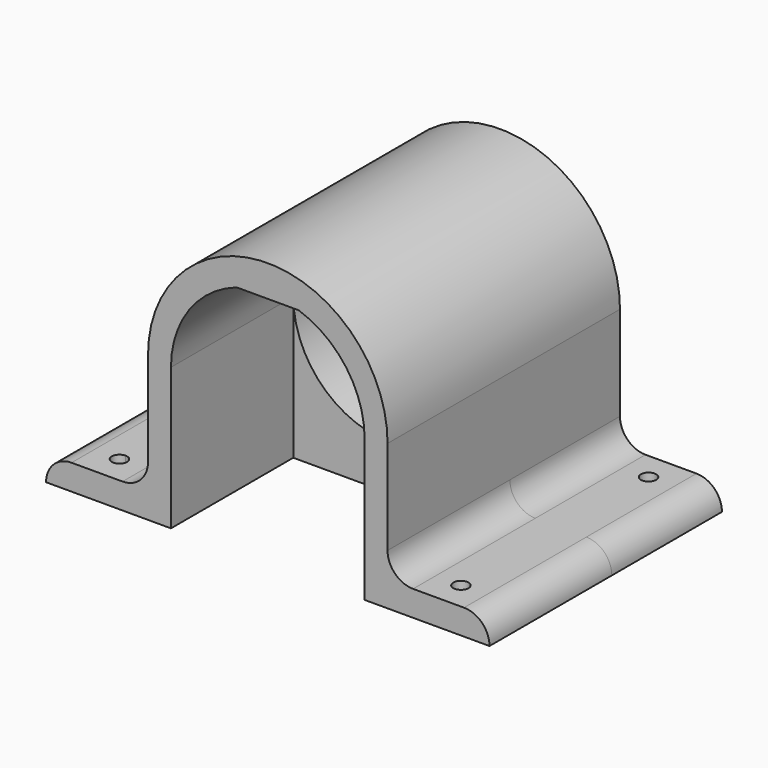
from build123d import *

# Parameters (mm, degrees)
F1_DEPTH  = 2
F2_R      = 1.5
F3_DEPTH  = 5
F4_R      = 19
F5_DEPTH  = 27
F6_W      = 47
F6_H      = 27
F7_DEPTH  = 5
F8_W      = 27
F8_H      = 5
F9_DEPTH  = 20
F10_W     = 27
F10_H     = 5
F11_DEPTH = 20
F12_R     = 4.99999
F14_DEPTH = 30
F16_DEPTH = 4
F18_DEPTH = 25


# Not quite as in the source:
# - a fillet or chamfer is up to 0.001 mm smaller than in the source, because OpenCascade refuses the exact size


with BuildPart() as f1:
    # F0 (on Front) → F1 (new body)
    with BuildSketch(Plane.XZ):
        with BuildLine():
            Line((-23.5, -23.5), (0, -23.5))
            Line((0, -23.5), (23.5, -23.5))
            Line((23.5, -23.5), (23.5, 0))
            ThreePointArc((23.5, 0), (0, 23.5), (-23.5, 0))
            Line((-23.5, 0), (-23.5, -23.5))
        make_face()
    extrude(amount=F1_DEPTH)

    # F2 (on face) → F3 (cut)
    with BuildSketch(Plane.XZ.offset(2)):
        with Locations((15.5, 0)):
            Circle(F2_R)
        with Locations((7.75, 13.4233937587)):
            Circle(F2_R)
        with Locations((-7.75, 13.4233937587)):
            Circle(F2_R)
        with Locations((-15.5, 0)):
            Circle(F2_R)
        with Locations((-7.75, -13.4233937587)):
            Circle(F2_R)
        with Locations((7.75, -13.4233937587)):
            Circle(F2_R)
        with BuildLine():
            Line((6.5, -7), (6.5, 7))
            ThreePointArc((6.5, 7), (0, 13.5), (-6.5, 7))
            Line((-6.5, 7), (-6.5, -7))
            ThreePointArc((-6.5, -7), (0, -13.5), (6.5, -7))
        make_face()
    extrude(amount=-F3_DEPTH, mode=Mode.SUBTRACT)

    # F4 (on Front) → F5 (join)
    with BuildSketch(Plane.XZ):
        with BuildLine():
            ThreePointArc((23.5, 0), (0, 23.5), (-23.5, 0))
            Line((-23.5, 0), (-23.5, -23.5))
            Line((-23.5, -23.5), (23.5, -23.5))
            Line((23.5, -23.5), (23.5, 0))
        make_face()
        with Locations((0, -0.6784388353)):
            Circle(F4_R, mode=Mode.SUBTRACT)
    extrude(amount=F5_DEPTH)

    # F6 (on face) → F7 (join)
    with BuildSketch(Plane(origin=(0, 0, -23.5), x_dir=(1, 0, 0), z_dir=(0, 0, -1))):
        with Locations((0, 13.5)):
            Rectangle(F6_W, F6_H)
    extrude(amount=F7_DEPTH)

    # F8 (on face) → F9 (join)
    with BuildSketch(Plane(origin=(-23.5, 0, 0), x_dir=(0, -1, 0), z_dir=(-1, 0, 0))):
        with Locations((13.5, -26)):
            Rectangle(F8_W, F8_H)
    extrude(amount=F9_DEPTH)

    # F10 (on face) → F11 (join)
    with BuildSketch(Plane.YZ.offset(23.5)):
        with Locations((-13.5, -26)):
            Rectangle(F10_W, F10_H)
    extrude(amount=F11_DEPTH)

    # F12 (radius 5 in the source; OpenCascade refuses exactly that, so slightly less here)
    f12_edges = [f1.edges().sort_by_distance(p)[0] for p in [
        (23.5, -13.5, -23.5),
        (43.5, -13.5, -23.5),
        (-23.5, -13.5, -23.5),
        (-43.5, -13.5, -23.5),
    ]]
    fillet(f12_edges, radius=F12_R)

    # F13 (on face) → F14 (join)
    with BuildSketch(Plane.XZ.offset(27)):
        with BuildLine():
            Line((23.5, -18.5), (23.5, 0))
            ThreePointArc((23.5, 0), (0, 23.5), (-23.5, 0))
            Line((-23.5, 0), (-23.5, -18.5))
            ThreePointArc((-23.5, -18.5), (-24.9644660941, -22.0355339059), (-28.5, -23.5))
            Line((-28.5, -23.5), (-38.5, -23.5))
            ThreePointArc((-38.5, -23.5), (-42.0355339059, -24.9644660941), (-43.5, -28.5))
            Line((-43.5, -28.5), (-19, -28.5))
            Line((-19, -28.5), (-19, -0.6784388353))
            ThreePointArc((-19, -0.6784388353), (0, 18.3215611647), (19, -0.6784388353))
            Line((19, -0.6784388353), (19, -28.5))
            Line((19, -28.5), (43.5, -28.5))
            ThreePointArc((43.5, -28.5), (42.0355339059, -24.9644660941), (38.5, -23.5))
            Line((38.5, -23.5), (28.5, -23.5))
            ThreePointArc((28.5, -23.5), (24.9644660941, -22.0355339059), (23.5, -18.5))
        make_face()
    extrude(amount=F14_DEPTH)

    # F15 (on face) → F16 (join)
    with BuildSketch(Plane.XZ.offset(57)):
        with BuildLine():
            ThreePointArc((6.0827625303, 17.3215611647), (3.0822070015, 18.0698944239), (0, 18.3215611647))
            Line((0, 18.3215611647), (0, 17.3215611647))
            Line((0, 17.3215611647), (6.0827625303, 17.3215611647))
        make_face()
        with BuildLine():
            Line((0, 17.3215611647), (0, 18.3215611647))
            ThreePointArc((0, 18.3215611647), (-3.0822070015, 18.0698944239), (-6.0827625303, 17.3215611647))
            Line((-6.0827625303, 17.3215611647), (0, 17.3215611647))
        make_face()
    extrude(amount=-F16_DEPTH)

    # F17 (on face) → F18 (cut)
    with BuildSketch(Plane(origin=(0, 0, -28.5), x_dir=(1, 0, 0), z_dir=(0, 0, -1))):
        with BuildLine():
            ThreePointArc((-35, 5.5), (-34.5606601718, 4.4393398282), (-33.5, 4))
            Line((-33.5, 4), (-33.5, 5.5))
            Line((-33.5, 5.5), (-35, 5.5))
        make_face()
        with BuildLine():
            ThreePointArc((35, 51.5), (33.5, 53), (32, 51.5))
            ThreePointArc((32, 51.5), (33.5, 50), (35, 51.5))
        make_face()
        with BuildLine():
            ThreePointArc((-33.5, 53), (-35, 51.5), (-33.5, 50))
            Line((-33.5, 50), (-33.5, 51.5))
            Line((-33.5, 51.5), (-33.5, 53))
        make_face()
        with BuildLine():
            Line((-33.5, 51.5), (-33.5, 50))
            ThreePointArc((-33.5, 50), (-32.4393398282, 50.4393398282), (-32, 51.5))
            Line((-32, 51.5), (-33.5, 51.5))
        make_face()
        with BuildLine():
            ThreePointArc((35, 5.5), (33.5, 7), (32, 5.5))
            ThreePointArc((32, 5.5), (33.5, 4), (35, 5.5))
        make_face()
        with BuildLine():
            Line((-33.5, 5.5), (-33.5, 4))
            ThreePointArc((-33.5, 4), (-32.4393398282, 4.4393398282), (-32, 5.5))
            Line((-32, 5.5), (-33.5, 5.5))
        make_face()
        with BuildLine():
            Line((-33.5, 7), (-33.5, 5.5))
            Line((-33.5, 5.5), (-32, 5.5))
            ThreePointArc((-32, 5.5), (-32.4393398282, 6.5606601718), (-33.5, 7))
        make_face()
        with BuildLine():
            Line((-35, 5.5), (-33.5, 5.5))
            Line((-33.5, 5.5), (-33.5, 7))
            ThreePointArc((-33.5, 7), (-34.5606601718, 6.5606601718), (-35, 5.5))
        make_face()
        with BuildLine():
            ThreePointArc((-32, 51.5), (-32.4393398282, 52.5606601718), (-33.5, 53))
            Line((-33.5, 53), (-33.5, 51.5))
            Line((-33.5, 51.5), (-32, 51.5))
        make_face()
    extrude(amount=-F18_DEPTH, mode=Mode.SUBTRACT)


solid = f1.part
